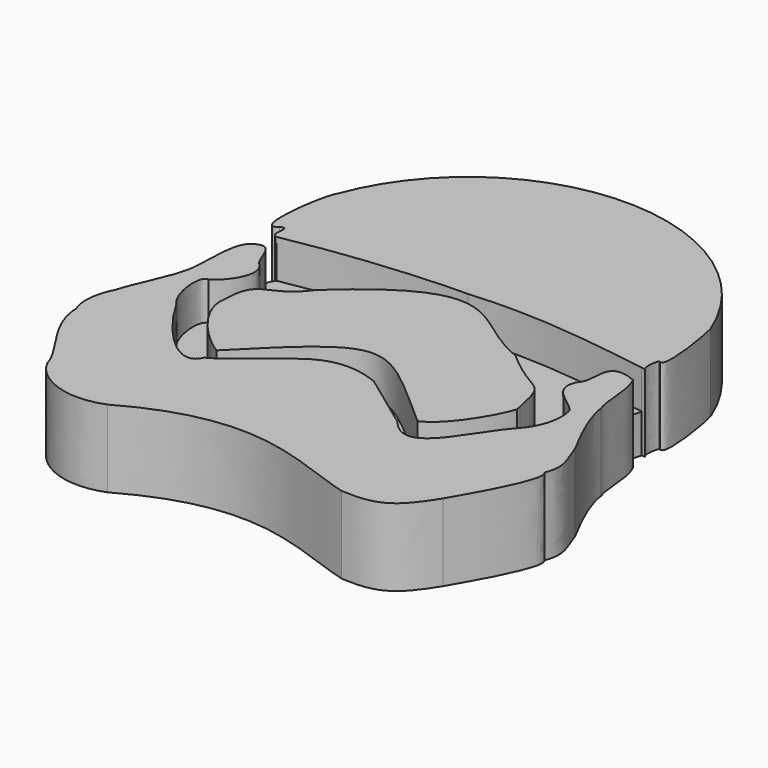
from build123d import *

# Parameters (mm, degrees)
F1_DEPTH = 10
F2_DEPTH = 5


with BuildPart() as f1:
    # F0 (on Top) → F1 (new body)
    with BuildSketch(Plane.XY):
        with BuildLine():
            add(Edge.make_bspline(
                [(-58.1226199865, -55.6246191263), (-63.2839827268, -57.6445940277), (-67.999497056, -54.5978136361), (-68.7818229198, -51.6151934862)],
                knots=[0, 0, 0, 0, 11.3883317978, 11.3883317978, 11.3883317978, 11.3883317978], degree=3))
            add(Edge.make_bspline(
                [(-58.1226199865, -55.6246191263), (-43.9918413758, -47.6057678461), (-35.4623011208, -53.5006423074), (-27.8376664372, -55.5990051041)],
                knots=[0, 0, 0, 0, 30.2849643811, 30.2849643811, 30.2849643811, 30.2849643811], degree=3))
            add(Edge.make_bspline(
                [(-27.8376664372, -55.5990051041), (-22.922385484, -55.9385158122), (-21.3960334659, -54.5720644295), (-18.810691312, -50.4905991256)],
                knots=[0, 0, 0, 0, 10.3721787273, 10.3721787273, 10.3721787273, 10.3721787273], degree=3))
            add(Edge.make_bspline(
                [(-18.810691312, -50.4905991256), (-16.8555881828, -47.0588095486), (-13.2214128971, -40.8080294728), (-14.3552748486, -39.6450944245)],
                knots=[0, 0, 0, 0, 11.725003543, 11.725003543, 11.725003543, 11.725003543], degree=3))
            add(Edge.make_bspline(
                [(-14.3552748486, -39.6450944245), (-13.358800672, -37.2957400978), (-14.499751851, -35.8436182141), (-15.2170648798, -33.6107686162)],
                knots=[0, 0, 0, 0, 6.0955532988, 6.0955532988, 6.0955532988, 6.0955532988], degree=3))
            add(Edge.make_bspline(
                [(-15.2170648798, -33.6107686162), (-15.5976144597, -32.8465029597), (-18.3635577559, -28.0061010271), (-18.6747275293, -25.0672847033)],
                knots=[0, 0, 0, 0, 9.2166451797, 9.2166451797, 9.2166451797, 9.2166451797], degree=3))
            add(Edge.make_bspline(
                [(-18.6747275293, -25.0672847033), (-19.3699859083, -23.2892837375), (-18.9244989306, -20.4473361373), (-20.0321637094, -18.2353835553)],
                knots=[0, 0, 0, 0, 6.9654509027, 6.9654509027, 6.9654509027, 6.9654509027], degree=3))
            add(Edge.make_bspline(
                [(-20.0321637094, -18.2353835553), (-20.3133088168, -18.1676502646), (-20.5373250575, -18.0838141171), (-20.7144234292, -17.9877220947)],
                knots=[0, 0, 0, 0, 0.3673031565, 0.3673031565, 0.3673031565, 0.3673031565], degree=3))
            add(Edge.make_bspline(
                [(-24.0373555571, -22.0555979759), (-22.7702460956, -20.8470092187), (-24.6360648495, -16.7431267564), (-20.7144234292, -17.9877220947)],
                knots=[0, 0, 0, 0, 5.253216019, 5.253216019, 5.253216019, 5.253216019], degree=3))
            add(Edge.make_bspline(
                [(-20.9948178381, -27.3108910769), (-22.0320466906, -25.9279180318), (-25.5586244166, -24.7523933649), (-24.0373555571, -22.0555979759)],
                knots=[0, 0, 0, 0, 6.0724905393, 6.0724905393, 6.0724905393, 6.0724905393], degree=3))
            add(Edge.make_bspline(
                [(-22.5029297736, -33.7363111501), (-19.5502133987, -30.472404399), (-20.9948178381, -26.7591356285), (-20.9948178381, -27.3108910769)],
                knots=[0.0171795738, 0.0171795738, 0.0171795738, 0.0171795738, 6.6300877223, 6.6300877223, 6.6300877223, 6.6300877223], degree=3))
            add(Edge.make_bspline(
                [(-22.5029297736, -33.7363111501), (-22.5099653948, -33.7447715347), (-22.5176605475, -33.7532460607), (-22.52603136, -33.7617397308)],
                knots=[4.5524467422, 4.5524467422, 4.5524467422, 4.5524467422, 4.6137139781, 4.6137139781, 4.6137139781, 4.6137139781], degree=3))
            add(Edge.make_bspline(
                [(-22.52603136, -33.7617397308), (-25.8356519043, -37.3118557036), (-28.6266990006, -45.5105565488), (-32.871413976, -40.2773432434)],
                knots=[0, 0, 0, 0, 12.226202624, 12.226202624, 12.226202624, 12.226202624], degree=3))
            add(Edge.make_bspline(
                [(-32.871413976, -40.2773432434), (-35.3388004005, -38.4646058083), (-37.5976525247, -36.7827527225), (-40.2735732496, -34.8391309381)],
                knots=[0, 0, 0, 0, 9.185102884, 9.185102884, 9.185102884, 9.185102884], degree=3))
            add(Edge.make_bspline(
                [(-48.1676608324, -34.983150661), (-44.8851175606, -33.0948606133), (-41.8309345841, -34.2770330608), (-40.2735732496, -34.8391309381)],
                knots=[0, 0, 0, 0, 7.8954012213, 7.8954012213, 7.8954012213, 7.8954012213], degree=3))
            add(Edge.make_bspline(
                [(-56.8860433996, -41.4402782917), (-56.2372282147, -41.5691547096), (-49.5927520096, -35.6062240899), (-48.1676608324, -34.983150661)],
                knots=[0, 0, 0, 0, 10.8491793158, 10.8491793158, 10.8491793158, 10.8491793158], degree=3))
            add(Edge.make_bspline(
                [(-66.4268657565, -34.1106206179), (-63.3403360844, -39.521433413), (-58.1652745605, -44.8127947748), (-56.8860433996, -41.4402782917)],
                knots=[0, 0, 0, 0, 12.0312581579, 12.0312581579, 12.0312581579, 12.0312581579], degree=3))
            add(Edge.make_bspline(
                [(-66.4268657565, -34.1106206179), (-68.154156208, -32.2895906866), (-68.4999004006, -27.7257822454), (-67.2552287579, -27.8640799224)],
                knots=[0, 0, 0, 0, 6.3012265411, 6.3012265411, 6.3012265411, 6.3012265411], degree=3))
            add(Edge.make_bspline(
                [(-67.2552287579, -27.8640799224), (-66.079698503, -27.3108910769), (-63.3137524128, -24.0609068424), (-65.3190612793, -22.0555979759)],
                knots=[0, 0, 0, 0, 6.1226797261, 6.1226797261, 6.1226797261, 6.1226797261], degree=3))
            add(Edge.make_bspline(
                [(-65.3190612793, -22.0555979759), (-66.411848294, -21.139873907), (-66.3668151268, -17.8011589419), (-68.4001393604, -18.8883112106)],
                knots=[0, 0, 0, 0, 4.2772194553, 4.2772194553, 4.2772194553, 4.2772194553], degree=3))
            add(Edge.make_bspline(
                [(-68.798519671, -19.1399119794), (-68.6411711893, -19.0477365072), (-68.5095729121, -18.9644036287), (-68.4001393604, -18.8883112106)],
                knots=[0, 0, 0, 0, 0.2259555121, 0.2259555121, 0.2259555121, 0.2259555121], degree=3))
            add(Edge.make_bspline(
                [(-70.067986846, -26.5247467905), (-69.8742344975, -22.745013237), (-70.0241699815, -20.1939307153), (-68.798519671, -19.1399119794)],
                knots=[0, 0, 0, 0, 7.493152347, 7.493152347, 7.493152347, 7.493152347], degree=3))
            add(Edge.make_bspline(
                [(-73.2250139117, -35.6281735003), (-72.3938569427, -32.6010882854), (-70.3005716205, -29.4030141085), (-70.067986846, -26.5247467905)],
                knots=[0, 0, 0, 0, 9.6353099459, 9.6353099459, 9.6353099459, 9.6353099459], degree=3))
            add(Edge.make_bspline(
                [(-73.7265050411, -41.1366224289), (-74.7283548117, -38.8358160853), (-73.4927356243, -36.0011607409), (-73.2250139117, -35.6281735003)],
                knots=[0, 0, 0, 0, 5.5312297866, 5.5312297866, 5.5312297866, 5.5312297866], degree=3))
            add(Edge.make_bspline(
                [(-68.7818229198, -51.6151934862), (-70.0163170695, -48.6725866795), (-73.5774710774, -45.4226061702), (-73.7265050411, -41.1366224289)],
                knots=[0, 0, 0, 0, 11.5866445826, 11.5866445826, 11.5866445826, 11.5866445826], degree=3))
        make_face()
        with BuildLine():
            add(Edge.make_bspline(
                [(-22.5029297736, -33.7363111501), (-22.5099653948, -33.7447715347), (-22.5176605475, -33.7532460607), (-22.52603136, -33.7617397308)],
                knots=[4.5524467422, 4.5524467422, 4.5524467422, 4.5524467422, 4.6137139781, 4.6137139781, 4.6137139781, 4.6137139781], degree=3))
            add(Edge.make_bspline(
                [(-22.52603136, -33.7617397308), (-22.5183010854, -33.7532666251), (-22.5106005908, -33.744790404), (-22.5029297736, -33.7363111501)],
                knots=[0, 0, 0, 0, 0.0171795738, 0.0171795738, 0.0171795738, 0.0171795738], degree=3))
        make_face()
    extrude(amount=F1_DEPTH)



with BuildPart() as f1b:
    # F0 (on Top) → F1, piece 2 (new body)
    with BuildSketch(Plane.XY):
        with BuildLine():
            add(Edge.make_bspline(
                [(-67.6843374968, -16.301067546), (-68.8070309462, -16.110695874), (-67.7085577487, -14.2640178157), (-68.444557246, -14.294838786)],
                knots=[0, 0, 0, 0, 1.9636063162, 1.9636063162, 1.9636063162, 1.9636063162], degree=3))
            add(Edge.make_bspline(
                [(-67.6843374968, -16.301067546), (-57.2978258133, -14.3109560013), (-48.1702126563, -13.96521274), (-44.7700001727, -13.9666104959)],
                knots=[0, 0, 0, 0, 23.0329447687, 23.0329447687, 23.0329447687, 23.0329447687], degree=3))
            add(Edge.make_bspline(
                [(-21.0256414992, -15.5816597024), (-27.8613186441, -14.5905211669), (-35.5955979866, -13.2222551257), (-44.7700001727, -13.9666104959)],
                knots=[0.5634156668, 0.5634156668, 0.5634156668, 0.5634156668, 24.2883608984, 24.2883608984, 24.2883608984, 24.2883608984], degree=3))
            add(Edge.make_bspline(
                [(-20.540157333, -15.6516004354), (-20.7014834487, -15.6285217719), (-20.8633090866, -15.6051970793), (-21.0256414992, -15.5816597024)],
                knots=[0, 0, 0, 0, 0.5634156668, 0.5634156668, 0.5634156668, 0.5634156668], degree=3))
            add(Edge.make_bspline(
                [(-20.540157333, -15.6516004354), (-20.9666647384, -15.530720117), (-20.7143625341, -13.6150686549), (-20.4928093114, -13.3934416105)],
                knots=[0, 0, 0, 0, 1.9269515682, 1.9269515682, 1.9269515682, 1.9269515682], degree=3))
            add(Edge.make_bspline(
                [(-68.444557246, -14.294838786), (-52.823425269, -9.8350617779), (-28.9938230357, -10.5042506711), (-20.4928093114, -13.3934416105)],
                knots=[0.3832242039, 0.3832242039, 0.3832242039, 0.3832242039, 48.2469231054, 48.2469231054, 48.2469231054, 48.2469231054], degree=3))
        make_face()
        with BuildLine():
            add(Edge.make_bspline(
                [(-68.444557246, -14.294838786), (-68.5372798978, -14.2987216719), (-68.6591182943, -14.332403193), (-68.8181817532, -14.4029492512)],
                knots=[1.9636063162, 1.9636063162, 1.9636063162, 1.9636063162, 2.2109852688, 2.2109852688, 2.2109852688, 2.2109852688], degree=3))
            add(Edge.make_bspline(
                [(-68.444557246, -14.294838786), (-52.823425269, -9.8350617779), (-28.9938230357, -10.5042506711), (-20.4928093114, -13.3934416105)],
                knots=[0.3832242039, 0.3832242039, 0.3832242039, 0.3832242039, 48.2469231054, 48.2469231054, 48.2469231054, 48.2469231054], degree=3))
            add(Edge.make_bspline(
                [(-20.4928093114, -13.3934416105), (-20.4580885299, -13.3587092599), (-20.4241229338, -13.3655816201), (-20.3936435282, -13.4274866432)],
                knots=[1.9269515682, 1.9269515682, 1.9269515682, 1.9269515682, 2.2289343767, 2.2289343767, 2.2289343767, 2.2289343767], degree=3))
            add(Edge.make_bspline(
                [(-20.9227539599, -4.5543652959), (-20.396463573, -6.3836588524), (-19.1319175065, -14.1633795574), (-20.3936435282, -13.4274866432)],
                knots=[0, 0, 0, 0, 8.8888829609, 8.8888829609, 8.8888829609, 8.8888829609], degree=3))
            ThreePointArc((-20.9227539599, -4.5543652959), (-45.051507143, 11.6693460001), (-68.8181817532, -5.0803022459))
            add(Edge.make_bspline(
                [(-68.8181817532, -5.0803022459), (-69.6757137775, -6.2863067724), (-71.1425766349, -16.6032444686), (-68.8181817532, -14.4029492512)],
                knots=[0, 0, 0, 0, 9.3226470053, 9.3226470053, 9.3226470053, 9.3226470053], degree=3))
        make_face()
    extrude(amount=F1_DEPTH)


with BuildPart() as f1c:
    # F0 (on Top) → F1, piece 3 (new body)
    with BuildSketch(Plane.XY):
        with BuildLine():
            add(Edge.make_bspline(
                [(-57.3563948274, -22.9075122625), (-42.3943921924, -9.0701039881), (-40.7593213022, -18.4597186744), (-32.6183512807, -21.5023010969)],
                knots=[0, 0, 0, 0, 24.7779219657, 24.7779219657, 24.7779219657, 24.7779219657], degree=3))
            add(Edge.make_bspline(
                [(-63.2718279958, -29.9373138696), (-63.1225630641, -24.5549082756), (-60.3111684322, -27.1474570036), (-57.3563948274, -22.9075122625)],
                knots=[0, 0, 0, 0, 9.1875165418, 9.1875165418, 9.1875165418, 9.1875165418], degree=3))
            add(Edge.make_bspline(
                [(-63.2718279958, -29.9373138696), (-63.2639022326, -30.256141622), (-63.2860429407, -30.6046057815), (-63.3421539318, -30.9599590962)],
                knots=[0, 0, 0, 0, 0.9635342565, 0.9635342565, 0.9635342565, 0.9635342565], degree=3))
            add(Edge.make_bspline(
                [(-56.9197532144, -39.4815085176), (-58.487649438, -38.6169751708), (-63.1408036747, -34.5851942183), (-63.3421539318, -30.9599590962)],
                knots=[0, 0, 0, 0, 10.4668973782, 10.4668973782, 10.4668973782, 10.4668973782], degree=3))
            add(Edge.make_bspline(
                [(-56.9197532144, -39.4815085176), (-43.9122989774, -26.2291021645), (-43.9122989774, -27.9352146684), (-31.3980240545, -38.8819330753)],
                knots=[0, 0, 0, 0, 25.5287710245, 25.5287710245, 25.5287710245, 25.5287710245], degree=3))
            add(Edge.make_bspline(
                [(-31.3980240545, -38.8819330753), (-28.5217368217, -37.6854320491), (-25.5750886347, -32.2533649556), (-25.1676890702, -30.5464928615)],
                knots=[0, 0, 0, 0, 9.0071253068, 9.0071253068, 9.0071253068, 9.0071253068], degree=3))
            add(Edge.make_bspline(
                [(-25.2421777695, -30.0322752446), (-25.2318782293, -30.2136114901), (-25.2062315585, -30.3847639148), (-25.1676890702, -30.5464928615)],
                knots=[0, 0, 0, 0, 0.3269633216, 0.3269633216, 0.3269633216, 0.3269633216], degree=3))
            add(Edge.make_bspline(
                [(-25.2421777695, -30.0322752446), (-26.5606287867, -23.7583834678), (-26.5024825931, -26.9564576447), (-32.6183512807, -21.5023010969)],
                knots=[0, 0, 0, 0, 11.276896498, 11.276896498, 11.276896498, 11.276896498], degree=3))
        make_face()
    extrude(amount=F1_DEPTH)


with BuildPart() as f1_1:
    add(f1.part)

    add(f1b.part)  # F2 merges F1b

    add(f1c.part)  # F2 merges F1c
    # F0 (on Top) → F2 (join)
    with BuildSketch(Plane.XY):
        with BuildLine():
            add(Edge.make_bspline(
                [(-24.0373555571, -22.0555979759), (-22.7702460956, -20.8470092187), (-24.6360648495, -16.7431267564), (-20.7144234292, -17.9877220947)],
                knots=[0, 0, 0, 0, 5.253216019, 5.253216019, 5.253216019, 5.253216019], degree=3))
            add(Edge.make_bspline(
                [(-20.7144234292, -17.9877220947), (-21.813576991, -17.3913310179), (-21.1054487195, -16.3228421967), (-21.0312174786, -15.7019669852)],
                knots=[0.3673031565, 0.3673031565, 0.3673031565, 0.3673031565, 2.6469546778, 2.6469546778, 2.6469546778, 2.6469546778], degree=3))
            Line((-21.0312174786, -15.7019669852), (-24.4916714728, -16.056895256))
            add(Edge.make_bspline(
                [(-24.4916714728, -16.056895256), (-24.387948215, -20.7935739309), (-27.0609576255, -25.7963631302), (-32.6183512807, -21.5023010969)],
                knots=[0, 0, 0, 0, 9.7824010075, 9.7824010075, 9.7824010075, 9.7824010075], degree=3))
            add(Edge.make_bspline(
                [(-25.2421777695, -30.0322752446), (-26.5606287867, -23.7583834678), (-26.5024825931, -26.9564576447), (-32.6183512807, -21.5023010969)],
                knots=[0, 0, 0, 0, 11.276896498, 11.276896498, 11.276896498, 11.276896498], degree=3))
            add(Edge.make_bspline(
                [(-25.1676890702, -30.5464928615), (-25.0874952957, -30.2105069454), (-25.1056902648, -30.0188618602), (-25.2421777695, -30.0322752446)],
                knots=[9.0071253068, 9.0071253068, 9.0071253068, 9.0071253068, 10.7801153614, 10.7801153614, 10.7801153614, 10.7801153614], degree=3))
            add(Edge.make_bspline(
                [(-25.1676890702, -30.5464928615), (-24.6695884139, -32.6365835158), (-22.0176965182, -33.1528147), (-22.5029297736, -33.7363111501)],
                knots=[0.3269633216, 0.3269633216, 0.3269633216, 0.3269633216, 4.5524467422, 4.5524467422, 4.5524467422, 4.5524467422], degree=3))
            add(Edge.make_bspline(
                [(-22.5029297736, -33.7363111501), (-19.5502133987, -30.472404399), (-20.9948178381, -26.7591356285), (-20.9948178381, -27.3108910769)],
                knots=[0.0171795738, 0.0171795738, 0.0171795738, 0.0171795738, 6.6300877223, 6.6300877223, 6.6300877223, 6.6300877223], degree=3))
            add(Edge.make_bspline(
                [(-20.9948178381, -27.3108910769), (-22.0320466906, -25.9279180318), (-25.5586244166, -24.7523933649), (-24.0373555571, -22.0555979759)],
                knots=[0, 0, 0, 0, 6.0724905393, 6.0724905393, 6.0724905393, 6.0724905393], degree=3))
        make_face()
        with BuildLine():
            add(Edge.make_bspline(
                [(-63.3421539318, -30.9599590962), (-63.5907090514, -32.5340693368), (-64.5058386941, -34.2433605353), (-66.4268657565, -34.1106206179)],
                knots=[0.9635342565, 0.9635342565, 0.9635342565, 0.9635342565, 5.2317064603, 5.2317064603, 5.2317064603, 5.2317064603], degree=3))
            add(Edge.make_bspline(
                [(-66.4268657565, -34.1106206179), (-63.3403360844, -39.521433413), (-58.1652745605, -44.8127947748), (-56.8860433996, -41.4402782917)],
                knots=[0, 0, 0, 0, 12.0312581579, 12.0312581579, 12.0312581579, 12.0312581579], degree=3))
            add(Edge.make_bspline(
                [(-56.8860433996, -41.4402782917), (-56.2372282147, -41.5691547096), (-49.5927520096, -35.6062240899), (-48.1676608324, -34.983150661)],
                knots=[0, 0, 0, 0, 10.8491793158, 10.8491793158, 10.8491793158, 10.8491793158], degree=3))
            add(Edge.make_bspline(
                [(-48.1676608324, -34.983150661), (-44.8851175606, -33.0948606133), (-41.8309345841, -34.2770330608), (-40.2735732496, -34.8391309381)],
                knots=[0, 0, 0, 0, 7.8954012213, 7.8954012213, 7.8954012213, 7.8954012213], degree=3))
            add(Edge.make_bspline(
                [(-32.871413976, -40.2773432434), (-35.3388004005, -38.4646058083), (-37.5976525247, -36.7827527225), (-40.2735732496, -34.8391309381)],
                knots=[0, 0, 0, 0, 9.185102884, 9.185102884, 9.185102884, 9.185102884], degree=3))
            add(Edge.make_bspline(
                [(-22.52603136, -33.7617397308), (-25.8356519043, -37.3118557036), (-28.6266990006, -45.5105565488), (-32.871413976, -40.2773432434)],
                knots=[0, 0, 0, 0, 12.226202624, 12.226202624, 12.226202624, 12.226202624], degree=3))
            add(Edge.make_bspline(
                [(-22.52603136, -33.7617397308), (-22.5183010854, -33.7532666251), (-22.5106005908, -33.744790404), (-22.5029297736, -33.7363111501)],
                knots=[0, 0, 0, 0, 0.0171795738, 0.0171795738, 0.0171795738, 0.0171795738], degree=3))
            add(Edge.make_bspline(
                [(-25.1676890702, -30.5464928615), (-24.6695884139, -32.6365835158), (-22.0176965182, -33.1528147), (-22.5029297736, -33.7363111501)],
                knots=[0.3269633216, 0.3269633216, 0.3269633216, 0.3269633216, 4.5524467422, 4.5524467422, 4.5524467422, 4.5524467422], degree=3))
            add(Edge.make_bspline(
                [(-31.3980240545, -38.8819330753), (-28.5217368217, -37.6854320491), (-25.5750886347, -32.2533649556), (-25.1676890702, -30.5464928615)],
                knots=[0, 0, 0, 0, 9.0071253068, 9.0071253068, 9.0071253068, 9.0071253068], degree=3))
            add(Edge.make_bspline(
                [(-56.9197532144, -39.4815085176), (-43.9122989774, -26.2291021645), (-43.9122989774, -27.9352146684), (-31.3980240545, -38.8819330753)],
                knots=[0, 0, 0, 0, 25.5287710245, 25.5287710245, 25.5287710245, 25.5287710245], degree=3))
            add(Edge.make_bspline(
                [(-56.9197532144, -39.4815085176), (-58.487649438, -38.6169751708), (-63.1408036747, -34.5851942183), (-63.3421539318, -30.9599590962)],
                knots=[0, 0, 0, 0, 10.4668973782, 10.4668973782, 10.4668973782, 10.4668973782], degree=3))
        make_face()
        with BuildLine():
            add(Edge.make_bspline(
                [(-68.4001393604, -18.8883112106), (-67.0325769991, -17.9374042413), (-69.1264453682, -18.1172287217), (-67.6843374968, -16.301067546)],
                knots=[0.2259555121, 0.2259555121, 0.2259555121, 0.2259555121, 3.0496622165, 3.0496622165, 3.0496622165, 3.0496622165], degree=3))
            add(Edge.make_bspline(
                [(-65.3190612793, -22.0555979759), (-66.411848294, -21.139873907), (-66.3668151268, -17.8011589419), (-68.4001393604, -18.8883112106)],
                knots=[0, 0, 0, 0, 4.2772194553, 4.2772194553, 4.2772194553, 4.2772194553], degree=3))
            add(Edge.make_bspline(
                [(-67.2552287579, -27.8640799224), (-66.079698503, -27.3108910769), (-63.3137524128, -24.0609068424), (-65.3190612793, -22.0555979759)],
                knots=[0, 0, 0, 0, 6.1226797261, 6.1226797261, 6.1226797261, 6.1226797261], degree=3))
            add(Edge.make_bspline(
                [(-66.4268657565, -34.1106206179), (-68.154156208, -32.2895906866), (-68.4999004006, -27.7257822454), (-67.2552287579, -27.8640799224)],
                knots=[0, 0, 0, 0, 6.3012265411, 6.3012265411, 6.3012265411, 6.3012265411], degree=3))
            add(Edge.make_bspline(
                [(-63.3421539318, -30.9599590962), (-63.5907090514, -32.5340693368), (-64.5058386941, -34.2433605353), (-66.4268657565, -34.1106206179)],
                knots=[0.9635342565, 0.9635342565, 0.9635342565, 0.9635342565, 5.2317064603, 5.2317064603, 5.2317064603, 5.2317064603], degree=3))
            add(Edge.make_bspline(
                [(-63.3421539318, -30.9599590962), (-63.3613494955, -30.6143502412), (-63.3400843587, -30.2724363219), (-63.2718279958, -29.9373138696)],
                knots=[10.4668973782, 10.4668973782, 10.4668973782, 10.4668973782, 11.4647505646, 11.4647505646, 11.4647505646, 11.4647505646], degree=3))
            add(Edge.make_bspline(
                [(-63.2718279958, -29.9373138696), (-63.1225630641, -24.5549082756), (-60.3111684322, -27.1474570036), (-57.3563948274, -22.9075122625)],
                knots=[0, 0, 0, 0, 9.1875165418, 9.1875165418, 9.1875165418, 9.1875165418], degree=3))
            add(Edge.make_bspline(
                [(-65.0932639837, -16.5277309716), (-64.6549612284, -18.5671057552), (-64.7363066673, -27.0280372351), (-57.3563948274, -22.9075122625)],
                knots=[0, 0, 0, 0, 10.0279984873, 10.0279984873, 10.0279984873, 10.0279984873], degree=3))
            Line((-65.0932639837, -16.5277309716), (-67.6843374968, -16.301067546))
        make_face()
        with BuildLine():
            add(Edge.make_bspline(
                [(-67.6843374968, -16.301067546), (-57.2978258133, -14.3109560013), (-48.1702126563, -13.96521274), (-44.7700001727, -13.9666104959)],
                knots=[0, 0, 0, 0, 23.0329447687, 23.0329447687, 23.0329447687, 23.0329447687], degree=3))
            Line((-67.6843374968, -16.301067546), (-65.0932639837, -16.5277309716))
            add(Edge.make_bspline(
                [(-65.0932639837, -16.5277309716), (-64.6549612284, -18.5671057552), (-64.7363066673, -27.0280372351), (-57.3563948274, -22.9075122625)],
                knots=[0, 0, 0, 0, 10.0279984873, 10.0279984873, 10.0279984873, 10.0279984873], degree=3))
            add(Edge.make_bspline(
                [(-57.3563948274, -22.9075122625), (-42.3943921924, -9.0701039881), (-40.7593213022, -18.4597186744), (-32.6183512807, -21.5023010969)],
                knots=[0, 0, 0, 0, 24.7779219657, 24.7779219657, 24.7779219657, 24.7779219657], degree=3))
            add(Edge.make_bspline(
                [(-24.4916714728, -16.056895256), (-24.387948215, -20.7935739309), (-27.0609576255, -25.7963631302), (-32.6183512807, -21.5023010969)],
                knots=[0, 0, 0, 0, 9.7824010075, 9.7824010075, 9.7824010075, 9.7824010075], degree=3))
            Line((-24.4916714728, -16.056895256), (-21.0312174786, -15.7019669852))
            add(Edge.make_bspline(
                [(-21.0312174786, -15.7019669852), (-21.0261631988, -15.6596926407), (-21.0240476771, -15.619493441), (-21.0256414927, -15.581659701)],
                knots=[2.6469546778, 2.6469546778, 2.6469546778, 2.6469546778, 2.8021722995, 2.8021722995, 2.8021722995, 2.8021722995], degree=3))
            add(Edge.make_bspline(
                [(-21.0256414992, -15.5816597024), (-27.8613186441, -14.5905211669), (-35.5955979866, -13.2222551257), (-44.7700001727, -13.9666104959)],
                knots=[0.5634156668, 0.5634156668, 0.5634156668, 0.5634156668, 24.2883608984, 24.2883608984, 24.2883608984, 24.2883608984], degree=3))
        make_face()
    extrude(amount=F2_DEPTH)


solid = f1_1.part
